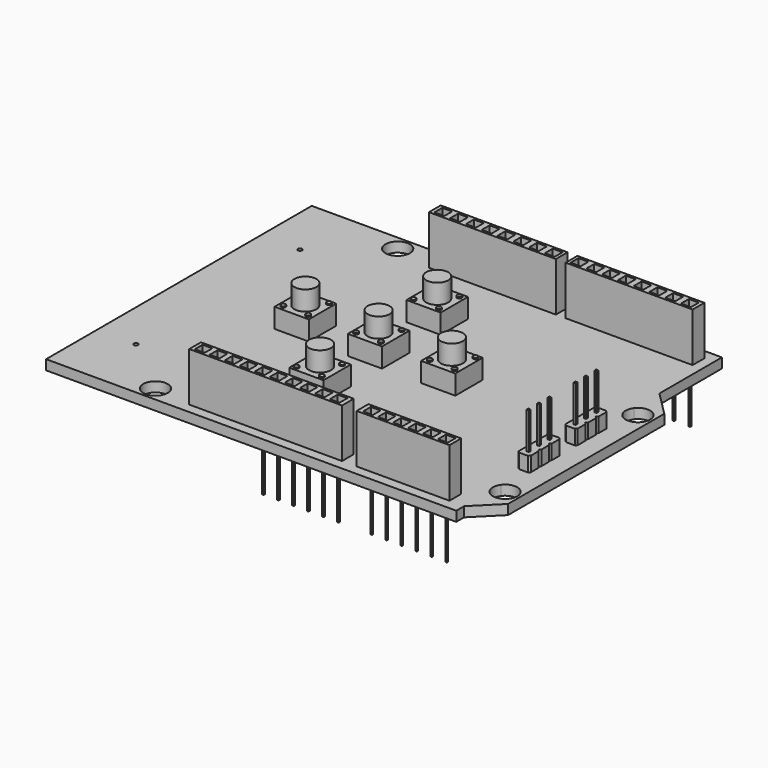
from build123d import *

# Parameters (mm, degrees)
F0_R      = 1.984375
F1_DEPTH  = 1.6002
F2_W      = 20.6375
F2_H      = 2.3876
F2_W_2    = 1.6002
F2_H_2    = 1.6002
F3_DEPTH  = 7.9502
F4_W      = 1.5875
F4_H      = 1.5875
F4_W_2    = 15.08125
F4_H_2    = 2.38125
F5_DEPTH  = 7.9502
F7_DEPTH  = 2.38125
F8_W      = 0.374374032
F8_H      = 0.3703085634
F9_DEPTH  = 5.953125
F10_W     = 5.55625
F10_H     = 5.55625
F11_DEPTH = 3.175
F12_R     = 1.7859375
F13_DEPTH = 3.175
F12_R_2   = 0.381
F14_DEPTH = 0.1984375
F15_W     = 0.2454817295
F15_H     = 0.2611353993
F16_DEPTH = 8.09625
F17_W     = 0.2549191635
F17_H     = 0.2452690575
F18_DEPTH = 8.09625
F19_R     = 0.3405237666
F19_R_2   = 0.3421588279
F20_DEPTH = 1.6002


# Not quite as in the source:
# - a length typed as a fraction of an inch, garbled in the dataset ("3 / 203.2 mm" for 3/8 in), is restored


with BuildPart() as f1:
    # F0 (on Top) → F1 (new body)
    with BuildSketch(Plane.XY):
        with BuildLine():
            Line((66.675, 0), (0, 0))
            Line((0, 0), (0, -53.975))
            Line((0, -53.975), (66.675, -53.975))
            Line((66.675, -53.975), (66.675, -52.3875))
            Line((66.675, -52.3875), (66.675, -47.228125))
            ThreePointArc((66.675, -47.228125), (66.278125, -46.0375), (66.675, -44.846875))
            Line((66.675, -44.846875), (66.675, -32.54375))
            Line((66.675, -32.54375), (66.675, -20.240625))
            ThreePointArc((66.675, -20.240625), (66.278125, -19.05), (66.675, -17.859375))
            Line((66.675, -17.859375), (66.675, -12.7))
            Line((66.675, -12.7), (66.675, 0))
        make_face()
        with Locations((15.875, -51.59375)):
            Circle(F0_R, mode=Mode.SUBTRACT)
        with Locations((15.875, -2.38125)):
            Circle(F0_R, mode=Mode.SUBTRACT)
        with BuildLine():
            Line((70.64375, -16.66875), (66.675, -12.7))
            Line((66.675, -12.7), (66.675, -17.859375))
            ThreePointArc((66.675, -17.859375), (68.8900144732, -17.1674565804), (70.246875, -19.05))
            ThreePointArc((70.246875, -19.05), (68.8900144732, -20.9325434196), (66.675, -20.240625))
            Line((66.675, -20.240625), (66.675, -32.54375))
            Line((66.675, -32.54375), (70.64375, -32.54375))
            Line((70.64375, -32.54375), (70.64375, -16.66875))
        make_face()
        with BuildLine():
            Line((66.675, -47.228125), (66.675, -52.3875))
            Line((66.675, -52.3875), (70.64375, -48.41875))
            Line((70.64375, -48.41875), (70.64375, -32.54375))
            Line((70.64375, -32.54375), (66.675, -32.54375))
            Line((66.675, -32.54375), (66.675, -44.846875))
            ThreePointArc((66.675, -44.846875), (68.8900144732, -44.1549565804), (70.246875, -46.0375))
            ThreePointArc((70.246875, -46.0375), (68.8900144732, -47.9200434196), (66.675, -47.228125))
        make_face()
    extrude(amount=F1_DEPTH)

    # F2 (on face) → F3 (join)
    with BuildSketch(Plane.XY.offset(1.6002)):
        with Locations((32.55645, -2.794)):
            Rectangle(F2_W, F2_H)
        with Locations((23.622, -2.8067)):
            Rectangle(F2_W_2, F2_H_2, mode=Mode.SUBTRACT)
        with Locations((26.1874, -2.8067)):
            Rectangle(F2_W_2, F2_H_2, mode=Mode.SUBTRACT)
        with Locations((28.7528, -2.8067)):
            Rectangle(F2_W_2, F2_H_2, mode=Mode.SUBTRACT)
        with Locations((31.3182, -2.8067)):
            Rectangle(F2_W_2, F2_H_2, mode=Mode.SUBTRACT)
        with Locations((33.8836, -2.8067)):
            Rectangle(F2_W_2, F2_H_2, mode=Mode.SUBTRACT)
        with Locations((36.449, -2.8067)):
            Rectangle(F2_W_2, F2_H_2, mode=Mode.SUBTRACT)
        with Locations((39.0144, -2.8067)):
            Rectangle(F2_W_2, F2_H_2, mode=Mode.SUBTRACT)
        with Locations((41.5798, -2.8067)):
            Rectangle(F2_W_2, F2_H_2, mode=Mode.SUBTRACT)
        with Locations((54.78145, -2.794)):
            Rectangle(F2_W, F2_H)
        with Locations((45.7581, -2.8067)):
            Rectangle(F2_W_2, F2_H_2, mode=Mode.SUBTRACT)
        with Locations((48.3235, -2.8067)):
            Rectangle(F2_W_2, F2_H_2, mode=Mode.SUBTRACT)
        with Locations((50.8889, -2.8067)):
            Rectangle(F2_W_2, F2_H_2, mode=Mode.SUBTRACT)
        with Locations((53.4543, -2.8067)):
            Rectangle(F2_W_2, F2_H_2, mode=Mode.SUBTRACT)
        with Locations((56.0197, -2.8067)):
            Rectangle(F2_W_2, F2_H_2, mode=Mode.SUBTRACT)
        with Locations((58.5851, -2.8067)):
            Rectangle(F2_W_2, F2_H_2, mode=Mode.SUBTRACT)
        with Locations((61.1505, -2.8067)):
            Rectangle(F2_W_2, F2_H_2, mode=Mode.SUBTRACT)
        with Locations((63.7159, -2.8067)):
            Rectangle(F2_W_2, F2_H_2, mode=Mode.SUBTRACT)
    extrude(amount=F3_DEPTH)

    # F4 (on face) → F5 (join)
    with BuildSketch(Plane.XY.offset(1.6002)):
        Polygon((46.8249, -49.99355), (31.74365, -49.99355), (21.9909958541, -49.99355), (21.9909958541, -52.3748), (31.74365, -52.3748), (46.8249, -52.3748), align=None)
        with Locations((23.3670595814, -51.184175)):
            Rectangle(F4_W, F4_H, mode=Mode.SUBTRACT)
        with Locations((25.7927595814, -51.184175)):
            Rectangle(F4_W, F4_H, mode=Mode.SUBTRACT)
        with Locations((28.2438595814, -51.184175)):
            Rectangle(F4_W, F4_H, mode=Mode.SUBTRACT)
        with Locations((30.6695595814, -51.184175)):
            Rectangle(F4_W, F4_H, mode=Mode.SUBTRACT)
        with Locations((33.1327125, -51.184175)):
            Rectangle(F4_W, F4_H, mode=Mode.SUBTRACT)
        with Locations((35.5584125, -51.184175)):
            Rectangle(F4_W, F4_H, mode=Mode.SUBTRACT)
        with Locations((38.0095125, -51.184175)):
            Rectangle(F4_W, F4_H, mode=Mode.SUBTRACT)
        with Locations((40.4352125, -51.184175)):
            Rectangle(F4_W, F4_H, mode=Mode.SUBTRACT)
        with Locations((42.8863125, -51.184175)):
            Rectangle(F4_W, F4_H, mode=Mode.SUBTRACT)
        with Locations((45.3120125, -51.184175)):
            Rectangle(F4_W, F4_H, mode=Mode.SUBTRACT)
        with Locations((56.746775, -51.184175)):
            Rectangle(F4_W_2, F4_H_2)
        with Locations((50.7190375, -51.184175)):
            Rectangle(F4_W, F4_H, mode=Mode.SUBTRACT)
        with Locations((53.1447375, -51.184175)):
            Rectangle(F4_W, F4_H, mode=Mode.SUBTRACT)
        with Locations((55.5958375, -51.184175)):
            Rectangle(F4_W, F4_H, mode=Mode.SUBTRACT)
        with Locations((58.0215375, -51.184175)):
            Rectangle(F4_W, F4_H, mode=Mode.SUBTRACT)
        with Locations((60.4726375, -51.184175)):
            Rectangle(F4_W, F4_H, mode=Mode.SUBTRACT)
        with Locations((62.8983375, -51.184175)):
            Rectangle(F4_W, F4_H, mode=Mode.SUBTRACT)
    extrude(amount=F5_DEPTH)

    # F6 (on face) → F7 (join)
    with BuildSketch(Plane.XY.offset(1.6002)):
        Polygon((67.2041666667, -33.7312), (65.7489583333, -33.7312), (65.484375, -33.9957833333), (65.484375, -35.5832833333), (65.7489583333, -35.8478666667), (65.484375, -36.11245), (65.484375, -37.69995), (65.7489583333, -37.9645333333), (65.484375, -38.2291166667), (65.484375, -39.8166166667), (65.7489583333, -40.0812), (67.2041666667, -40.0812), (67.46875, -39.8166166667), (67.46875, -38.2291166667), (67.2041666667, -37.9645333333), (67.46875, -37.69995), (67.46875, -36.11245), (67.2041666667, -35.8478666667), (67.46875, -35.5832833333), (67.46875, -33.9957833333), align=None)
        Polygon((67.2041666667, -24.2062), (65.7489583333, -24.2062), (65.484375, -24.4707833333), (65.484375, -26.0582833333), (65.7489583333, -26.3228666667), (65.484375, -26.58745), (65.484375, -28.17495), (65.7489583333, -28.4395333333), (65.484375, -28.7041166667), (65.484375, -30.2916166667), (65.7489583333, -30.5562), (67.2041666667, -30.5562), (67.46875, -30.2916166667), (67.46875, -28.7041166667), (67.2041666667, -28.4395333333), (67.46875, -28.17495), (67.46875, -26.58745), (67.2041666667, -26.3228666667), (67.46875, -26.0582833333), (67.46875, -24.4707833333), align=None)
    extrude(amount=F7_DEPTH)

    # F8 (on face) → F9 (join)
    with BuildSketch(Plane.XY.offset(3.98145)):
        with Locations((66.4765625, -25.2645333333)):
            Rectangle(F8_W, F8_H)
        with Locations((66.4765625, -27.3812)):
            Rectangle(F8_W, F8_H)
        with Locations((66.4765625, -29.4978666667)):
            Rectangle(F8_W, F8_H)
        with Locations((66.4765625, -34.7895333333)):
            Rectangle(F8_W, F8_H)
        with Locations((66.4765625, -36.9062)):
            Rectangle(F8_W, F8_H)
        with Locations((66.4765625, -39.0228666667)):
            Rectangle(F8_W, F8_H)
    extrude(amount=F9_DEPTH)

    # F10 (on face) → F11 (join)
    with BuildSketch(Plane.XY.offset(1.6002)):
        with Locations((20.240625, -26.590625)):
            Rectangle(F10_W, F10_H)
        with Locations((32.146875, -14.684375)):
            Rectangle(F10_W, F10_H)
        with Locations((32.146875, -26.590625)):
            Rectangle(F10_W, F10_H)
        with Locations((44.053125, -26.590625)):
            Rectangle(F10_W, F10_H)
        with Locations((32.146875, -38.496875)):
            Rectangle(F10_W, F10_H)
    extrude(amount=F11_DEPTH)

    # F12 (on face) → F13 (join)
    with BuildSketch(Plane.XY.offset(4.7752)):
        with Locations((20.240625, -26.590625)):
            Circle(F12_R)
        with Locations((32.146875, -26.590625)):
            Circle(F12_R)
        with Locations((32.146875, -14.684375)):
            Circle(F12_R)
        with Locations((44.053125, -26.590625)):
            Circle(F12_R)
        with Locations((32.146875, -38.496875)):
            Circle(F12_R)
    extrude(amount=F13_DEPTH)

    # F12 (on face) → F14 (join)
    with BuildSketch(Plane.XY.offset(4.7752)):
        with Locations((18.25625, -28.60053)):
            Circle(F12_R_2)
        with Locations((18.2204839615, -24.4197200538)):
            Circle(F12_R_2)
        with Locations((22.3460539615, -24.4197200538)):
            Circle(F12_R_2)
        with Locations((22.29324, -28.575)):
            Circle(F12_R_2)
        with Locations((30.09426, -28.575)):
            Circle(F12_R_2)
        with Locations((30.0414460385, -24.4197200538)):
            Circle(F12_R_2)
        with Locations((34.1670160385, -24.4197200538)):
            Circle(F12_R_2)
        with Locations((34.13125, -28.60053)):
            Circle(F12_R_2)
        with Locations((30.09426, -36.5125)):
            Circle(F12_R_2)
        with Locations((30.0414460385, -40.6677799462)):
            Circle(F12_R_2)
        with Locations((34.1670160385, -40.6677799462)):
            Circle(F12_R_2)
        with Locations((34.13125, -36.48697)):
            Circle(F12_R_2)
        with Locations((42.06875, -28.60053)):
            Circle(F12_R_2)
        with Locations((42.0329839615, -24.4197200538)):
            Circle(F12_R_2)
        with Locations((46.1585539615, -24.4197200538)):
            Circle(F12_R_2)
        with Locations((46.10574, -28.575)):
            Circle(F12_R_2)
        with Locations((34.1670160385, -16.8552799462)):
            Circle(F12_R_2)
        with Locations((30.0414460385, -16.8552799462)):
            Circle(F12_R_2)
        with Locations((30.09426, -12.7)):
            Circle(F12_R_2)
        with Locations((34.13125, -12.67447)):
            Circle(F12_R_2)
    extrude(amount=F14_DEPTH)

    # F15 (on face) → F16 (join)
    with BuildSketch(Plane(origin=(0, 0, 0), x_dir=(1, 0, 0), z_dir=(0, 0, -1))):
        with Locations((33.1366687918, 51.1983409524)):
            Rectangle(F15_W, F15_H)
        with Locations((35.5567323314, 51.1983409524)):
            Rectangle(F15_W, F15_H)
        with Locations((38.0111926686, 51.1983409524)):
            Rectangle(F15_W, F15_H)
        with Locations((40.4312562082, 51.1983409524)):
            Rectangle(F15_W, F15_H)
        with Locations((42.8902687918, 51.1983409524)):
            Rectangle(F15_W, F15_H)
        with Locations((45.3103323314, 51.1983409524)):
            Rectangle(F15_W, F15_H)
        with Locations((50.7207176686, 51.1983409524)):
            Rectangle(F15_W, F15_H)
        with Locations((53.1407812082, 51.1983409524)):
            Rectangle(F15_W, F15_H)
        with Locations((55.5997937918, 51.1983409524)):
            Rectangle(F15_W, F15_H)
        with Locations((58.0198573314, 51.1983409524)):
            Rectangle(F15_W, F15_H)
        with Locations((60.4743176686, 51.1983409524)):
            Rectangle(F15_W, F15_H)
        with Locations((62.8943812082, 51.1983409524)):
            Rectangle(F15_W, F15_H)
    extrude(amount=F16_DEPTH)

    # F17 (on face) → F18 (join)
    with BuildSketch(Plane(origin=(0, 0, 0), x_dir=(1, 0, 0), z_dir=(0, 0, -1))):
        with Locations((63.7159, 2.8067)):
            Rectangle(F17_W, F17_H)
        with Locations((61.1505, 2.8067)):
            Rectangle(F17_W, F17_H)
        with Locations((58.5851, 2.8067)):
            Rectangle(F17_W, F17_H)
        with Locations((56.0197, 2.8067)):
            Rectangle(F17_W, F17_H)
        with Locations((53.4543, 2.8067)):
            Rectangle(F17_W, F17_H)
        with Locations((50.8889, 2.8067)):
            Rectangle(F17_W, F17_H)
        with Locations((48.3235, 2.8067)):
            Rectangle(F17_W, F17_H)
        with Locations((45.7581, 2.8067)):
            Rectangle(F17_W, F17_H)
        with Locations((41.5798, 2.8067)):
            Rectangle(F17_W, F17_H)
        with Locations((39.0144, 2.8067)):
            Rectangle(F17_W, F17_H)
        with Locations((36.449, 2.8067)):
            Rectangle(F17_W, F17_H)
        with Locations((33.8836, 2.8067)):
            Rectangle(F17_W, F17_H)
        with Locations((31.3182, 2.8067)):
            Rectangle(F17_W, F17_H)
        with Locations((28.7528, 2.8067)):
            Rectangle(F17_W, F17_H)
        with Locations((26.1874, 2.8067)):
            Rectangle(F17_W, F17_H)
        with Locations((23.622, 2.8067)):
            Rectangle(F17_W, F17_H)
    extrude(amount=F18_DEPTH)

    # F19 (on face) → F20 (cut)
    with BuildSketch(Plane.XY.offset(1.6002)):
        with Locations((6.35, -43.65625)):
            Circle(F19_R)
        with Locations((6.35, -10.31875)):
            Circle(F19_R_2)
    extrude(amount=-F20_DEPTH, mode=Mode.SUBTRACT)


solid = f1.part
